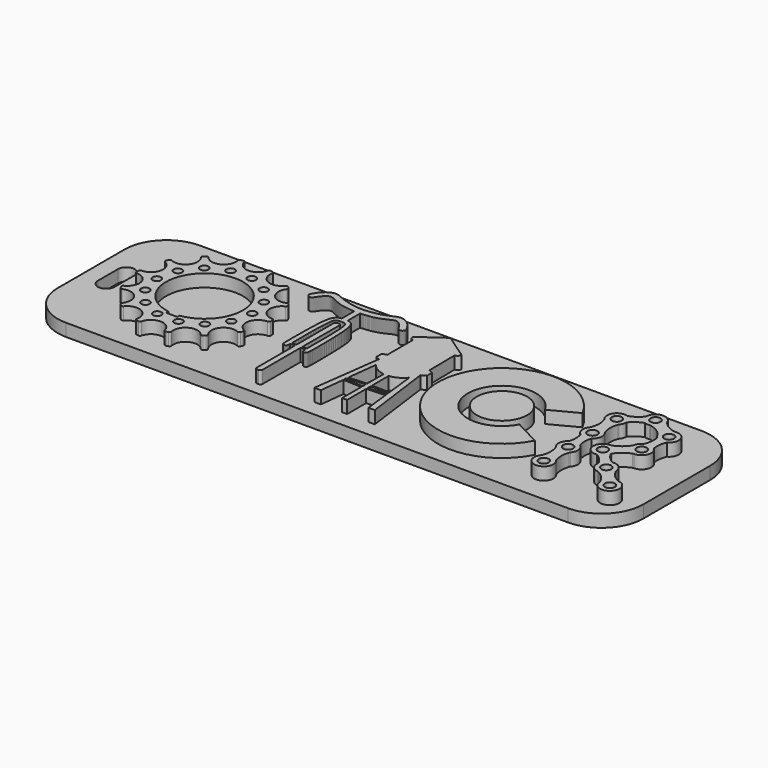
from build123d import *

# Parameters (mm, degrees)
F0_R     = 0.7946644
F1_DEPTH = 2.38125
F0_R_2   = 4.775327
F0_R_3   = 0.9406128
F2_W     = 111.125
F2_H     = 31.75
F3_DEPTH = 2.38125
F4_R     = 7.9375


# Not quite as in the source:
# - ends of sketch curves that miss each other by under 0.0002 mm in the source are joined


with BuildPart() as f1:
    # F0 (on Top) → F1 (new body)
    with BuildSketch(Plane.XY):
        with BuildLine():
            ThreePointArc((-33.590121634, 12.3507484588), (-33.6294176049, 12.5881754555), (-33.8237599562, 12.7301148883))
            ThreePointArc((-33.8237599562, 12.7301148883), (-34.0524121873, 12.7845207856), (-34.2820284084, 12.8347024108))
            ThreePointArc((-34.2820284084, 12.8347024108), (-34.5186909947, 12.7911373675), (-34.6571006347, 12.5942839271))
            ThreePointArc((-34.6571006347, 12.5942839271), (-36.8834641683, 10.8196634), (-39.1098143955, 12.5942824563))
            ThreePointArc((-39.1098143955, 12.5942824563), (-39.2482176053, 12.7911373675), (-39.4848817783, 12.8347100044))
            ThreePointArc((-39.4848817783, 12.8347100044), (-39.7145096927, 12.7845235519), (-39.9431718443, 12.7301060129))
            ThreePointArc((-39.9431718443, 12.7301060129), (-40.1374959801, 12.588167361), (-40.1767882188, 12.3507539588))
            ThreePointArc((-40.1767882188, 12.3507539588), (-41.4126795487, 9.7859172011), (-44.1885186964, 10.4188115386))
            ThreePointArc((-44.1885186964, 10.4188115386), (-44.3986514992, 10.5361025158), (-44.6307849214, 10.4726580069))
            ThreePointArc((-44.6307849214, 10.4726580069), (-44.8158899503, 10.3278331325), (-44.9982810167, 10.1796047146))
            ThreePointArc((-44.9982810167, 10.1796047146), (-45.1117808241, 9.9673948786), (-45.0441752505, 9.7364351367))
            ThreePointArc((-45.0441752505, 9.7364351367), (-45.0448396583, 6.8893584849), (-47.8203948412, 6.2551970986))
            ThreePointArc((-47.8203948412, 6.2551970986), (-48.0606127411, 6.2697127824), (-48.242238874, 6.1118337222))
            ThreePointArc((-48.242238874, 6.1118337222), (-48.3461595976, 5.9010204757), (-48.4461774197, 5.6883278976))
            ThreePointArc((-48.4461774197, 5.6883278976), (-48.4563582226, 5.4478968636), (-48.2952461097, 5.2691472525))
            ThreePointArc((-48.2952461097, 5.2691472525), (-47.0605440786, 2.7037326004), (-49.2860584001, 0.9280908492))
            ThreePointArc((-49.2860584001, 0.9280908492), (-49.5087779976, 0.8369447193), (-49.6039106856, 0.6158986702))
            ThreePointArc((-49.6039106856, 0.6158986702), (-49.6060984, 0.380873), (-49.6039273899, 0.1458470219))
            ThreePointArc((-49.6039273899, 0.1458470219), (-49.5087779976, -0.0751987193), (-49.2860584, -0.1663445635))
            ThreePointArc((-49.2860584, -0.1663445635), (-47.0605440786, -1.9419866004), (-48.2952490252, -4.507395207))
            ThreePointArc((-48.2952490252, -4.507395207), (-48.4563582226, -4.6861508636), (-48.4461664662, -4.9265768698))
            ThreePointArc((-48.4461664662, -4.9265768698), (-48.3461595976, -5.1392744757), (-48.2422297671, -5.3500831279))
            ThreePointArc((-48.2422297671, -5.3500831279), (-48.0606127411, -5.5079667824), (-47.8203983996, -5.4934437005))
            ThreePointArc((-47.8203983996, -5.4934437005), (-45.0448396583, -6.1276124849), (-45.0441705492, -8.9746928823))
            ThreePointArc((-45.0441705492, -8.9746928823), (-45.1117808241, -9.2056488786), (-44.9982729443, -9.4178489662))
            ThreePointArc((-44.9982729443, -9.4178489662), (-44.8158899503, -9.5660871325), (-44.6307918654, -9.7109210511))
            ThreePointArc((-44.6307918654, -9.7109210511), (-44.3986514992, -9.7743565158), (-44.1885265788, -9.6570592469))
            ThreePointArc((-44.1885265788, -9.6570592469), (-41.4126773347, -9.0241468673), (-40.1767873331, -11.5890081606))
            ThreePointArc((-40.1767873331, -11.5890081606), (-40.1374959801, -11.826421361), (-39.9431725738, -11.9683629594))
            ThreePointArc((-39.9431725738, -11.9683629594), (-39.7145096927, -12.0227775519), (-39.4848812536, -12.0729614947))
            ThreePointArc((-39.4848812536, -12.0729614947), (-39.2482176053, -12.0293913675), (-39.1098079653, -11.8325379271))
            ThreePointArc((-39.1098079653, -11.8325379271), (-36.8834641683, -10.0579174), (-34.6571183418, -11.8325419771))
            ThreePointArc((-34.6571183418, -11.8325419771), (-34.5186909947, -12.0293913675), (-34.2820268217, -12.0729640044))
            ThreePointArc((-34.2820268217, -12.0729640044), (-34.0524121873, -12.0227747856), (-33.8237621557, -11.9683600129))
            ThreePointArc((-33.8237621557, -11.9683600129), (-33.6294176049, -11.8264294555), (-33.590121634, -11.5890024588))
            ThreePointArc((-33.590121634, -11.5890024588), (-32.3542358625, -9.0241490812), (-29.5783874048, -9.657043269))
            ThreePointArc((-29.5783874048, -9.657043269), (-29.3682749652, -9.77435434), (-29.1361396594, -9.7109242752))
            ThreePointArc((-29.1361396594, -9.7109242752), (-28.9510364024, -9.566081034), (-28.7686379166, -9.4178462371))
            ThreePointArc((-28.7686379166, -9.4178462371), (-28.6551277759, -9.2056488786), (-28.7227333495, -8.9746891367))
            ThreePointArc((-28.7227333495, -8.9746891367), (-28.7220760775, -6.1276214327), (-25.9465343862, -5.4934411767))
            ThreePointArc((-25.9465343862, -5.4934411767), (-25.7063158426, -5.5079649417), (-25.5246899728, -5.3500775075))
            ThreePointArc((-25.5246899728, -5.3500775075), (-25.4207696215, -5.1392645481), (-25.32075216, -4.9265722676))
            ThreePointArc((-25.32075216, -4.9265722676), (-25.3105542527, -4.6861401007), (-25.4716830986, -4.5073913165))
            ThreePointArc((-25.4716830986, -4.5073913165), (-26.7063870953, -1.9419742188), (-24.4808501999, -0.1663448374))
            ThreePointArc((-24.4808501999, -0.1663448374), (-24.2581307695, -0.0751988834), (-24.162997923, 0.1458468613))
            ThreePointArc((-24.162997923, 0.1458468613), (-24.1608356, 0.380873), (-24.1630066101, 0.6158989781))
            ThreePointArc((-24.1630066101, 0.6158989781), (-24.2581307695, 0.8369448834), (-24.4808502, 0.9280905635))
            ThreePointArc((-24.4808502, 0.9280905635), (-26.7063870953, 2.7037202188), (-25.4716849748, 5.269141207))
            ThreePointArc((-25.4716849748, 5.269141207), (-25.3105542527, 5.4478861007), (-25.3207421338, 5.6883228698))
            ThreePointArc((-25.3207421338, 5.6883228698), (-25.4207696215, 5.9010105481), (-25.524699079, 6.1118189129))
            ThreePointArc((-25.524699079, 6.1118189129), (-25.7063158426, 6.2697109417), (-25.9465356004, 6.2551897005))
            ThreePointArc((-25.9465356004, 6.2551897005), (-28.7220760775, 6.8893674327), (-28.7227380508, 9.7364388823))
            ThreePointArc((-28.7227380508, 9.7364388823), (-28.6551277759, 9.9673948786), (-28.7686356557, 10.1795949662))
            ThreePointArc((-28.7686356557, 10.1795949662), (-28.9510364024, 10.327827034), (-29.1361421346, 10.4726670511))
            ThreePointArc((-29.1361421346, 10.4726670511), (-29.3682749652, 10.53610034), (-29.5783919067, 10.4187928628))
            ThreePointArc((-29.5783919067, 10.4187928628), (-32.3542336486, 9.785919415), (-33.590121634, 12.3507484588))
        make_face()
        with Locations((-38.8217918, -8.4056474)):
            Circle(F0_R, mode=Mode.SUBTRACT)
        with Locations((-42.4421554, -6.6945002)):
            Circle(F0_R, mode=Mode.SUBTRACT)
        with Locations((-34.8175072, -8.3765136)):
            Circle(F0_R, mode=Mode.SUBTRACT)
        with Locations((-31.2224166, -6.61289)):
            Circle(F0_R, mode=Mode.SUBTRACT)
        with Locations((-44.961556, -3.5819842)):
            Circle(F0_R, mode=Mode.SUBTRACT)
        with Locations((-28.7485582, -3.464052)):
            Circle(F0_R, mode=Mode.SUBTRACT)
        with Locations((-45.8809852, 0.3154172)):
            Circle(F0_R, mode=Mode.SUBTRACT)
        with BuildLine():
            ThreePointArc((-37.9286029944, -6.8447817713), (-36.883467, 7.681722), (-35.8383310056, -6.8447817713))
            Line((-35.8383310056, -6.8447817713), (-35.8383332, -7.3637648))
            Line((-35.8383332, -7.3637648), (-37.9286008, -7.3637648))
            Line((-37.9286008, -7.3637648), (-37.9286029944, -6.8447817713))
        make_face(mode=Mode.SUBTRACT)
        with Locations((-27.8859234, 0.4463288)):
            Circle(F0_R, mode=Mode.SUBTRACT)
        with Locations((-45.0183504, 4.225798)):
            Circle(F0_R, mode=Mode.SUBTRACT)
        with Locations((-28.8053526, 4.3437302)):
            Circle(F0_R, mode=Mode.SUBTRACT)
        with Locations((-42.544492, 7.374636)):
            Circle(F0_R, mode=Mode.SUBTRACT)
        with Locations((-38.9494014, 9.1382596)):
            Circle(F0_R, mode=Mode.SUBTRACT)
        with Locations((-31.3247532, 7.4562462)):
            Circle(F0_R, mode=Mode.SUBTRACT)
        with Locations((-34.9451168, 9.1673934)):
            Circle(F0_R, mode=Mode.SUBTRACT)
    extrude(amount=F1_DEPTH)



with BuildPart() as f1b:
    # F0 (on Top) → F1, piece 2 (new body)
    with BuildSketch(Plane.XY):
        with Locations((19.5524374, 0.380873)):
            Circle(F0_R_2)
    extrude(amount=F1_DEPTH)


with BuildPart() as f1c:
    # F0 (on Top) → F1, piece 3 (new body)
    with BuildSketch(Plane.XY):
        with BuildLine():
            ThreePointArc((25.2826844358, -2.633348701), (13.0777742, 0.380873), (25.2826844358, 3.395094701))
            Line((25.2826844358, 3.395094701), (30.3119282, 6.0406026))
            ThreePointArc((30.3119282, 6.0406026), (7.3951592, 0.380873), (30.3119366377, -5.2788610384))
            Line((30.3119366377, -5.2788610384), (25.2826844358, -2.633348701))
        make_face()
    extrude(amount=F1_DEPTH)


with BuildPart() as f1d:
    # F0 (on Top) → F1, piece 4 (new body)
    with BuildSketch(Plane.XY):
        with BuildLine():
            Line((4.4645834, -12.4356114), (5.679186, -12.4356114))
            Line((5.679186, -12.4356114), (3.958463, 0.54991))
            ThreePointArc((3.958463, 0.54991), (4.4173192561, 0.7397615753), (4.8236809314, 1.0251781026))
            Line((4.8236809314, 1.0251781026), (4.8493426, 2.198497))
            ThreePointArc((4.8493426, 2.198497), (4.4533409594, 2.4265248649), (4.0170864794, 2.5625312363))
            Line((4.0170864794, 2.5625312363), (3.941191, 8.6607142))
            ThreePointArc((3.941191, 8.6607142), (4.4449083132, 8.8954168394), (4.7161825983, 9.380420758))
            Line((4.7161825983, 9.380420758), (-0.0563372, 12.6585726))
            Line((-0.0563372, 12.6585726), (-4.574159, 9.4512384))
            ThreePointArc((-4.574159, 9.4512384), (-4.4374640474, 8.9238193385), (-3.9651421172, 8.6522138729))
            Line((-3.9651421172, 8.6522138729), (-3.959479, 2.5776174))
            ThreePointArc((-3.959479, 2.5776174), (-4.4068158157, 2.4445470258), (-4.8173908735, 2.2226291598))
            Line((-4.8173908735, 2.2226291598), (-4.7921164, 1.0034524))
            ThreePointArc((-4.7921164, 1.0034524), (-4.4323052844, 0.8270572106), (-4.0505879444, 0.7051075587))
            Line((-4.0505879444, 0.7051075587), (-5.7918858, -12.4356114))
            Line((-5.7918858, -12.4356114), (-4.5598334, -12.4356114))
            Line((-4.5598334, -12.4356114), (-4.0266874, -7.7761592))
            Line((-4.0266874, -7.7761592), (-0.5179314, -7.8915768))
            Line((-0.5179314, -7.8915768), (-0.5179314, -12.4356114))
            Line((-0.5179314, -12.4356114), (0.4226814, -12.4356114))
            Line((0.4226814, -12.4356114), (0.4226814, -7.9140812))
            Line((0.4226814, -7.9140812), (3.9224204, -7.6973938))
            Line((3.9224204, -7.6973938), (4.4645834, -12.4356114))
        make_face()
        Polygon((-0.5179314, -6.8287392), (-0.5179314, -7.5406758), (-4.0517318, -7.4238612), (-3.9769542, -7.088886), align=None, mode=Mode.SUBTRACT)
        with BuildLine():
            Line((-0.5179314, -6.4943736), (-3.9253668, -6.7382136))
            Line((-3.9253668, -6.7382136), (-3.2671258, -0.985393))
            ThreePointArc((-3.2671258, -0.985393), (-2.0560803671, -2.0688932492), (-0.5179318251, -2.5930131115))
            Line((-0.5179318251, -2.5930131115), (-0.5179314, -6.4943736))
        make_face(mode=Mode.SUBTRACT)
        Polygon((3.7990018, -7.0056756), (3.8354254, -7.323963), (0.4226814, -7.5932538), (0.4226814, -6.895592), align=None, mode=Mode.SUBTRACT)
        with BuildLine():
            Line((3.1691326, -1.1139932), (3.8027356, -6.6512186))
            Line((3.8027356, -6.6512186), (0.4226814, -6.5249552))
            Line((0.4226814, -6.5249552), (0.4226814, -2.6042874))
            ThreePointArc((0.4226814, -2.6042874), (1.9444372298, -2.1328635042), (3.1691326, -1.1139932))
        make_face(mode=Mode.SUBTRACT)
    extrude(amount=F1_DEPTH)


with BuildPart() as f1e:
    # F0 (on Top) → F1, piece 5 (new body)
    with BuildSketch(Plane.XY):
        with BuildLine():
            Line((-15.9458914, 11.6212112), (-15.9545528, 11.6212112))
            Line((-15.9545528, 11.6212112), (-16.547592, 11.655298))
            Line((-16.547592, 11.655298), (-17.088739, 11.705336))
            Line((-17.088739, 11.705336), (-17.581626, 11.768836))
            Line((-17.581626, 11.768836), (-18.0299106, 11.8433596))
            Line((-18.0299106, 11.8433596), (-18.437225, 11.9264938))
            Line((-18.437225, 11.9264938), (-18.8072268, 12.0157748))
            Line((-18.8072268, 12.0157748), (-19.1435482, 12.1087896))
            Line((-19.1435482, 12.1087896), (-19.4498214, 12.203049))
            Line((-19.4498214, 12.203049), (-19.7293738, 12.2964194))
            Line((-19.7293738, 12.2964194), (-19.9841612, 12.3877832))
            Line((-19.9841612, 12.3877832), (-20.215733, 12.4762514))
            Line((-20.215733, 12.4762514), (-20.4257656, 12.5610112))
            Line((-20.4257656, 12.5610112), (-20.6158338, 12.641199))
            Line((-20.6158338, 12.641199), (-20.7875378, 12.7159258))
            Line((-20.7875378, 12.7159258), (-20.9425286, 12.7843788))
            Line((-20.9425286, 12.7843788), (-21.082381, 12.8456944))
            Line((-21.082381, 12.8456944), (-21.2086952, 12.8992376))
            Line((-21.2086952, 12.8992376), (-21.3230968, 12.9454148))
            Line((-21.3230968, 12.9454148), (-21.4272114, 12.9848102))
            Line((-21.4272114, 12.9848102), (-21.5226392, 13.0180334))
            Line((-21.5226392, 13.0180334), (-21.6109804, 13.0457194))
            Line((-21.6109804, 13.0457194), (-21.6938606, 13.0684524))
            Line((-21.6938606, 13.0684524), (-21.77288, 13.0868674))
            Line((-21.77288, 13.0868674), (-21.8496388, 13.1015232))
            Line((-21.8496388, 13.1015232), (-21.925534, 13.1129786))
            Line((-21.925534, 13.1129786), (-22.001099, 13.1212844))
            Line((-22.001099, 13.1212844), (-22.0765878, 13.126339))
            Line((-22.0765878, 13.126339), (-22.1522798, 13.1281424))
            Line((-22.1522798, 13.1281424), (-22.2284544, 13.1266184))
            Line((-22.2284544, 13.1266184), (-22.3054418, 13.1216908))
            Line((-22.3054418, 13.1216908), (-22.3834706, 13.1133596))
            Line((-22.3834706, 13.1133596), (-22.4628456, 13.1015232))
            Line((-22.4628456, 13.1015232), (-22.54377, 13.0861562))
            Line((-22.54377, 13.0861562), (-22.6261168, 13.067157))
            Line((-22.6261168, 13.067157), (-22.7096828, 13.044424))
            Line((-22.7096828, 13.044424), (-22.7942648, 13.0178556))
            Line((-22.7942648, 13.0178556), (-22.8796596, 12.9873502))
            Line((-22.8796596, 12.9873502), (-22.9656894, 12.9528316))
            Line((-22.9656894, 12.9528316), (-23.0521002, 12.9141982))
            Line((-23.0521002, 12.9141982), (-23.1387142, 12.8713484))
            Line((-23.1387142, 12.8713484), (-23.2253536, 12.8242314))
            Line((-23.2253536, 12.8242314), (-23.3117898, 12.7730504))
            Line((-23.3117898, 12.7730504), (-23.3978196, 12.7180594))
            Line((-23.3978196, 12.7180594), (-23.4832906, 12.6595124))
            Line((-23.4832906, 12.6595124), (-23.5679996, 12.5976634))
            Line((-23.5679996, 12.5976634), (-23.6517688, 12.5327664))
            Line((-23.6517688, 12.5327664), (-23.7343696, 12.4650754))
            Line((-23.7343696, 12.4650754), (-23.8156242, 12.3948444))
            Line((-23.8156242, 12.3948444), (-23.895431, 12.322175))
            Line((-23.895431, 12.322175), (-23.9741456, 12.246483))
            Line((-23.9741456, 12.246483), (-24.0521744, 12.1670572))
            Line((-24.0521744, 12.1670572), (-24.1298984, 12.0832372))
            Line((-24.1298984, 12.0832372), (-24.2077494, 11.994261))
            Line((-24.2077494, 11.994261), (-24.2861846, 11.8994174))
            Line((-24.2861846, 11.8994174), (-24.3655596, 11.7980206))
            Line((-24.3655596, 11.7980206), (-24.446357, 11.689334))
            Line((-24.446357, 11.689334), (-24.5286022, 11.5731798))
            Line((-24.5286022, 11.5731798), (-24.610949, 11.4514884))
            Line((-24.610949, 11.4514884), (-24.6917718, 11.3267236))
            Line((-24.6917718, 11.3267236), (-24.7693688, 11.2014))
            Line((-24.7693688, 11.2014), (-24.842089, 11.0779052))
            Line((-24.842089, 11.0779052), (-24.9082052, 10.9587792))
            Line((-24.9082052, 10.9587792), (-24.9660664, 10.846435))
            Line((-24.9660664, 10.846435), (-25.0140216, 10.7433872))
            Line((-25.0140216, 10.7433872), (-25.0508008, 10.6514138))
            Line((-25.0508008, 10.6514138), (-25.0768866, 10.5699052))
            Line((-25.0768866, 10.5699052), (-25.093168, 10.4975406))
            Line((-25.093168, 10.4975406), (-25.1005848, 10.4329992))
            Line((-25.1005848, 10.4329992), (-25.100026, 10.3750364))
            Line((-25.100026, 10.3750364), (-25.092406, 10.3222806))
            Line((-25.092406, 10.3222806), (-25.0786138, 10.2735126))
            Line((-25.0786138, 10.2735126), (-25.0595892, 10.2273608))
            Line((-25.0595892, 10.2273608), (-25.0361196, 10.18286))
            Line((-25.0361196, 10.18286), (-25.0086368, 10.1401118))
            Line((-25.0086368, 10.1401118), (-24.977471, 10.0994718))
            Line((-24.977471, 10.0994718), (-24.942927, 10.0613718))
            Line((-24.942927, 10.0613718), (-24.9053858, 10.0261928))
            Line((-24.9053858, 10.0261928), (-24.8651522, 9.9943158))
            Line((-24.8651522, 9.9943158), (-24.822531, 9.9661218))
            Line((-24.822531, 9.9661218), (-24.7778778, 9.9420426))
            Line((-24.7778778, 9.9420426), (-24.7315482, 9.9223576))
            Line((-24.7315482, 9.9223576), (-24.6839232, 9.9069652))
            Line((-24.6839232, 9.9069652), (-24.6354346, 9.8957638))
            Line((-24.6354346, 9.8957638), (-24.5865396, 9.8885502))
            Line((-24.5865396, 9.8885502), (-24.5376446, 9.885172))
            Line((-24.5376446, 9.885172), (-24.489156, 9.8854768))
            Line((-24.489156, 9.8854768), (-24.441531, 9.8893122))
            Line((-24.441531, 9.8893122), (-24.3952014, 9.8965258))
            Line((-24.3952014, 9.8965258), (-24.3504466, 9.907016))
            Line((-24.3504466, 9.907016), (-24.3070888, 9.9211638))
            Line((-24.3070888, 9.9211638), (-24.2647978, 9.9393756))
            Line((-24.2647978, 9.9393756), (-24.2233196, 9.9621594))
            Line((-24.2233196, 9.9621594), (-24.1822732, 9.9898962))
            Line((-24.1822732, 9.9898962), (-24.1413792, 10.0230686))
            Line((-24.1413792, 10.0230686), (-24.1003328, 10.0621084))
            Line((-24.1003328, 10.0621084), (-24.0588292, 10.1074728))
            Line((-24.0588292, 10.1074728), (-24.0165128, 10.1594412))
            Line((-24.0165128, 10.1594412), (-23.9730026, 10.2177088))
            Line((-23.9730026, 10.2177088), (-23.927943, 10.2818184))
            Line((-23.927943, 10.2818184), (-23.8808768, 10.3513382))
            Line((-23.8808768, 10.3513382), (-23.831423, 10.425811))
            Line((-23.831423, 10.425811), (-23.7791752, 10.5047542))
            Line((-23.7791752, 10.5047542), (-23.7237524, 10.587736))
            Line((-23.7237524, 10.587736), (-23.6647482, 10.6743246))
            Line((-23.6647482, 10.6743246), (-23.6019086, 10.7639104))
            Line((-23.6019086, 10.7639104), (-23.5355638, 10.8555536))
            Line((-23.5355638, 10.8555536), (-23.466171, 10.9481366))
            Line((-23.466171, 10.9481366), (-23.3942382, 11.0405418))
            Line((-23.3942382, 11.0405418), (-23.3202734, 11.1317278))
            Line((-23.3202734, 11.1317278), (-23.244683, 11.220577))
            Line((-23.244683, 11.220577), (-23.1680258, 11.3059718))
            Line((-23.1680258, 11.3059718), (-23.0907082, 11.3868708))
            Line((-23.0907082, 11.3868708), (-23.0132636, 11.4622834))
            Line((-23.0132636, 11.4622834), (-22.936073, 11.531981))
            Line((-22.936073, 11.531981), (-22.859492, 11.5957858))
            Line((-22.859492, 11.5957858), (-22.7839524, 11.6535962))
            Line((-22.7839524, 11.6535962), (-22.7098606, 11.7052852))
            Line((-22.7098606, 11.7052852), (-22.6375722, 11.7507512))
            Line((-22.6375722, 11.7507512), (-22.5674682, 11.7898418))
            Line((-22.5674682, 11.7898418), (-22.4999804, 11.82243))
            Line((-22.4999804, 11.82243), (-22.4353374, 11.8485158))
            Line((-22.4353374, 11.8485158), (-22.3732598, 11.8685056))
            Line((-22.3732598, 11.8685056), (-22.3132904, 11.882882))
            Line((-22.3132904, 11.882882), (-22.2550228, 11.892153))
            Line((-22.2550228, 11.892153), (-22.1979744, 11.896852))
            Line((-22.1979744, 11.896852), (-22.1417388, 11.8974616))
            Line((-22.1417388, 11.8974616), (-22.0858842, 11.8944898))
            Line((-22.0858842, 11.8944898), (-22.0299788, 11.8884446))
            Line((-22.0299788, 11.8884446), (-21.9734384, 11.879707))
            Line((-21.9734384, 11.879707), (-21.915247, 11.8679214))
            Line((-21.915247, 11.8679214), (-21.8542616, 11.8527068))
            Line((-21.8542616, 11.8527068), (-21.7892884, 11.8335298))
            Line((-21.7892884, 11.8335298), (-21.7191844, 11.8100094))
            Line((-21.7191844, 11.8100094), (-21.6428066, 11.7816376))
            Line((-21.6428066, 11.7816376), (-21.5589866, 11.7479826))
            Line((-21.5589866, 11.7479826), (-21.4665814, 11.7086126))
            Line((-21.4665814, 11.7086126), (-21.3648036, 11.6632736))
            Line((-21.3648036, 11.6632736), (-21.2544152, 11.6127022))
            Line((-21.2544152, 11.6127022), (-21.13661, 11.5578382))
            Line((-21.13661, 11.5578382), (-21.012531, 11.4996468))
            Line((-21.012531, 11.4996468), (-20.8832958, 11.4390678))
            Line((-20.8832958, 11.4390678), (-20.7500982, 11.3770664))
            Line((-20.7500982, 11.3770664), (-20.6141066, 11.3145824))
            Line((-20.6141066, 11.3145824), (-20.476464, 11.2525556))
            Line((-20.476464, 11.2525556), (-20.3380848, 11.1918242))
            Line((-20.3380848, 11.1918242), (-20.1990706, 11.1327184))
            Line((-20.1990706, 11.1327184), (-20.059269, 11.0754414))
            Line((-20.059269, 11.0754414), (-19.9185022, 11.020171))
            Line((-19.9185022, 11.020171), (-19.7766686, 10.9671358))
            Line((-19.7766686, 10.9671358), (-19.6336158, 10.9164882))
            Line((-19.6336158, 10.9164882), (-19.489166, 10.8684568))
            Line((-19.489166, 10.8684568), (-19.3431922, 10.8232194))
            Line((-19.3431922, 10.8232194), (-19.1953388, 10.7809284))
            Line((-19.1953388, 10.7809284), (-19.0444628, 10.741406))
            Line((-19.0444628, 10.741406), (-18.8891926, 10.7044236))
            Line((-18.8891926, 10.7044236), (-18.7282328, 10.669778))
            Line((-18.7282328, 10.669778), (-18.560161, 10.6372152))
            Line((-18.560161, 10.6372152), (-18.3836564, 10.606532))
            Line((-18.3836564, 10.606532), (-18.1973982, 10.577449))
            Line((-18.1973982, 10.577449), (-17.9999894, 10.5497884))
            Line((-17.9999894, 10.5497884), (-17.7913538, 10.5234486))
            Line((-17.7913538, 10.5234486), (-17.5765206, 10.4987852))
            Line((-17.5765206, 10.4987852), (-17.3617382, 10.4763316))
            Line((-17.3617382, 10.4763316), (-17.1533058, 10.4565958))
            Line((-17.1533058, 10.4565958), (-16.9574464, 10.4400858))
            Line((-16.9574464, 10.4400858), (-16.7804846, 10.4273096))
            Line((-16.7804846, 10.4273096), (-16.6286688, 10.418826))
            Line((-16.6286688, 10.418826), (-16.5082728, 10.4150922))
            Line((-16.5082728, 10.4150922), (-16.5082728, 7.4820272))
            Line((-16.5082728, 7.4820272), (-16.7950134, 7.4200004))
            Line((-16.7950134, 7.4200004), (-16.8914318, 7.39267))
            Line((-16.8914318, 7.39267), (-16.9828464, 7.3597262))
            Line((-16.9828464, 7.3597262), (-17.0701462, 7.3207118))
            Line((-17.0701462, 7.3207118), (-17.1541948, 7.2752458))
            Line((-17.1541948, 7.2752458), (-17.235805, 7.2228456))
            Line((-17.235805, 7.2228456), (-17.315688, 7.1629778))
            Line((-17.315688, 7.1629778), (-17.3937168, 7.0945248))
            Line((-17.3937168, 7.0945248), (-17.4696374, 7.0162166))
            Line((-17.4696374, 7.0162166), (-17.5430942, 6.9267578))
            Line((-17.5430942, 6.9267578), (-17.6138586, 6.8249292))
            Line((-17.6138586, 6.8249292), (-17.6816258, 6.7094354))
            Line((-17.6816258, 6.7094354), (-17.746091, 6.5790318))
            Line((-17.746091, 6.5790318), (-17.8069494, 6.4324484))
            Line((-17.8069494, 6.4324484), (-17.8639978, 6.2680596))
            Line((-17.8639978, 6.2680596), (-17.9172108, 6.0828428))
            Line((-17.9172108, 6.0828428), (-17.9666392, 5.8734452))
            Line((-17.9666392, 5.8734452), (-18.0123592, 5.636514))
            Line((-18.0123592, 5.636514), (-18.0544216, 5.368671))
            Line((-18.0544216, 5.368671), (-18.0928518, 5.066538))
            Line((-18.0928518, 5.066538), (-18.1277006, 4.7267622))
            Line((-18.1277006, 4.7267622), (-18.1590696, 4.3459908))
            Line((-18.1590696, 4.3459908), (-18.1869842, 3.922395))
            Line((-18.1869842, 3.922395), (-18.2116476, 3.4605722))
            Line((-18.2116476, 3.4605722), (-18.2332884, 2.9666692))
            Line((-18.2332884, 2.9666692), (-18.2521098, 2.446782))
            Line((-18.2521098, 2.446782), (-18.2683404, 1.9070574))
            Line((-18.2683404, 1.9070574), (-18.2822088, 1.3536676))
            Line((-18.2822088, 1.3536676), (-18.2938928, 0.792734))
            Line((-18.2938928, 0.792734), (-18.3036464, 0.230378))
            Line((-18.3036464, 0.230378), (-18.3115966, -0.3270504))
            Line((-18.3115966, -0.3270504), (-18.3177434, -0.8723884))
            Line((-18.3177434, -0.8723884), (-18.3219598, -1.3982954))
            Line((-18.3219598, -1.3982954), (-18.3241188, -1.8974308))
            Line((-18.3241188, -1.8974308), (-18.3241696, -2.3624286))
            Line((-18.3241696, -2.3624286), (-18.3219852, -2.7859482))
            Line((-18.3219852, -2.7859482), (-18.317464, -3.1605982))
            Line((-18.317464, -3.1605982), (-18.3105044, -3.4790888))
            Line((-18.3105044, -3.4790888), (-18.3010302, -3.7365178))
            Line((-18.3010302, -3.7365178), (-18.2889398, -3.938016))
            Line((-18.2889398, -3.938016), (-18.274157, -4.0912542))
            Line((-18.274157, -4.0912542), (-18.2566056, -4.2038016))
            Line((-18.2566056, -4.2038016), (-18.2362348, -4.283329))
            Line((-18.2362348, -4.283329), (-18.2129684, -4.3374564))
            Line((-18.2129684, -4.3374564), (-18.1866794, -4.3737784))
            Line((-18.1866794, -4.3737784), (-18.1573678, -4.3999404))
            Line((-18.1573678, -4.3999404), (-18.1249828, -4.4222924))
            Line((-18.1249828, -4.4222924), (-18.08988, -4.4420536))
            Line((-18.08988, -4.4420536), (-18.0524912, -4.4591224))
            Line((-18.0524912, -4.4591224), (-18.0132228, -4.4734226))
            Line((-18.0132228, -4.4734226), (-17.9725066, -4.484878))
            Line((-17.9725066, -4.484878), (-17.9307744, -4.4934632))
            Line((-17.9307744, -4.4934632), (-17.888458, -4.4990258))
            Line((-17.888458, -4.4990258), (-17.8459384, -4.5015404))
            Line((-17.8459384, -4.5015404), (-17.803622, -4.5009562))
            Line((-17.803622, -4.5009562), (-17.7618136, -4.4972732))
            Line((-17.7618136, -4.4972732), (-17.7207672, -4.4905422))
            Line((-17.7207672, -4.4905422), (-17.6807114, -4.480814))
            Line((-17.6807114, -4.480814), (-17.641951, -4.4681394))
            Line((-17.641951, -4.4681394), (-17.6046892, -4.4525438))
            Line((-17.6046892, -4.4525438), (-17.5692308, -4.434078))
            Line((-17.5692308, -4.434078), (-17.535779, -4.4128182))
            Line((-17.535779, -4.4128182), (-17.5046386, -4.3870118))
            Line((-17.5046386, -4.3870118), (-17.4760382, -4.3478958))
            Line((-17.4760382, -4.3478958), (-17.4502572, -4.2850054))
            Line((-17.4502572, -4.2850054), (-17.427575, -4.1877742))
            Line((-17.427575, -4.1877742), (-17.4081948, -4.0456866))
            Line((-17.4081948, -4.0456866), (-17.3924214, -3.8482524))
            Line((-17.3924214, -3.8482524), (-17.385538, -3.6964874))
            Line((-17.385538, -3.6964874), (-16.5025578, -3.6964874))
            Line((-16.5025578, -3.6964874), (-16.5025578, -12.681331))
            ThreePointArc((-16.5025578, -12.681331), (-16.3716718103, -12.9972564103), (-16.0557464, -13.128117))
            Line((-16.0557464, -13.128117), (-15.9502094, -13.128117))
            Line((-15.9502094, -13.128117), (-15.8446724, -13.128117))
            ThreePointArc((-15.8446724, -13.128117), (-15.5287469897, -12.9972564103), (-15.3978864, -12.681331))
            Line((-15.3978864, -12.681331), (-15.3978864, -3.6964874))
            Line((-15.3978864, -3.6964874), (-14.5149062, -3.6964874))
            Line((-14.5149062, -3.6964874), (-14.5080228, -3.8482524))
            Line((-14.5080228, -3.8482524), (-14.4922494, -4.0456866))
            Line((-14.4922494, -4.0456866), (-14.4728692, -4.1877742))
            Line((-14.4728692, -4.1877742), (-14.4501616, -4.2850054))
            Line((-14.4501616, -4.2850054), (-14.4243806, -4.3478958))
            Line((-14.4243806, -4.3478958), (-14.3958056, -4.3870118))
            Line((-14.3958056, -4.3870118), (-14.3646398, -4.4128182))
            Line((-14.3646398, -4.4128182), (-14.3312134, -4.434078))
            Line((-14.3312134, -4.434078), (-14.2957296, -4.4525438))
            Line((-14.2957296, -4.4525438), (-14.2584932, -4.4681394))
            Line((-14.2584932, -4.4681394), (-14.2197074, -4.480814))
            Line((-14.2197074, -4.480814), (-14.179677, -4.4905422))
            Line((-14.179677, -4.4905422), (-14.1386052, -4.4972732))
            Line((-14.1386052, -4.4972732), (-14.0968222, -4.5009562))
            Line((-14.0968222, -4.5009562), (-14.0545058, -4.5015404))
            Line((-14.0545058, -4.5015404), (-14.0119862, -4.4990258))
            Line((-14.0119862, -4.4990258), (-13.9696444, -4.4934632))
            Line((-13.9696444, -4.4934632), (-13.9279122, -4.484878))
            Line((-13.9279122, -4.484878), (-13.887196, -4.4734226))
            Line((-13.887196, -4.4734226), (-13.847953, -4.4591224))
            Line((-13.847953, -4.4591224), (-13.8105642, -4.4420536))
            Line((-13.8105642, -4.4420536), (-13.7754614, -4.4222924))
            Line((-13.7754614, -4.4222924), (-13.7430764, -4.3999404))
            Line((-13.7430764, -4.3999404), (-13.7137394, -4.3737784))
            Line((-13.7137394, -4.3737784), (-13.6874758, -4.3374564))
            Line((-13.6874758, -4.3374564), (-13.664184, -4.283329))
            Line((-13.664184, -4.283329), (-13.6438132, -4.2038016))
            Line((-13.6438132, -4.2038016), (-13.6262872, -4.0912542))
            Line((-13.6262872, -4.0912542), (-13.6115044, -3.938016))
            Line((-13.6115044, -3.938016), (-13.599414, -3.7365178))
            Line((-13.599414, -3.7365178), (-13.5899398, -3.4790888))
            Line((-13.5899398, -3.4790888), (-13.5829802, -3.1605982))
            Line((-13.5829802, -3.1605982), (-13.578459, -2.7859482))
            Line((-13.578459, -2.7859482), (-13.5762746, -2.3624286))
            Line((-13.5762746, -2.3624286), (-13.5763, -1.8974308))
            Line((-13.5763, -1.8974308), (-13.5784844, -1.3982954))
            Line((-13.5784844, -1.3982954), (-13.5827008, -0.8723884))
            Line((-13.5827008, -0.8723884), (-13.5888222, -0.3270504))
            Line((-13.5888222, -0.3270504), (-13.5967978, 0.230378))
            Line((-13.5967978, 0.230378), (-13.606526, 0.792734))
            Line((-13.606526, 0.792734), (-13.6182354, 1.3536676))
            Line((-13.6182354, 1.3536676), (-13.6320784, 1.9070574))
            Line((-13.6320784, 1.9070574), (-13.648309, 2.446782))
            Line((-13.648309, 2.446782), (-13.6671558, 2.9666692))
            Line((-13.6671558, 2.9666692), (-13.6887966, 3.4605722))
            Line((-13.6887966, 3.4605722), (-13.71346, 3.922395))
            Line((-13.71346, 3.922395), (-13.7413746, 4.3459908))
            Line((-13.7413746, 4.3459908), (-13.7727182, 4.7267622))
            Line((-13.7727182, 4.7267622), (-13.8075924, 5.066538))
            Line((-13.8075924, 5.066538), (-13.8460226, 5.368671))
            Line((-13.8460226, 5.368671), (-13.8880596, 5.636514))
            Line((-13.8880596, 5.636514), (-13.9337796, 5.8734452))
            Line((-13.9337796, 5.8734452), (-13.9832334, 6.0828428))
            Line((-13.9832334, 6.0828428), (-14.0364464, 6.2680596))
            Line((-14.0364464, 6.2680596), (-14.0934948, 6.4324484))
            Line((-14.0934948, 6.4324484), (-14.1543532, 6.5790318))
            Line((-14.1543532, 6.5790318), (-14.2188184, 6.7094354))
            Line((-14.2188184, 6.7094354), (-14.2865602, 6.8249292))
            Line((-14.2865602, 6.8249292), (-14.3573246, 6.9267578))
            Line((-14.3573246, 6.9267578), (-14.4308068, 7.0162166))
            Line((-14.4308068, 7.0162166), (-14.506702, 7.0945248))
            Line((-14.506702, 7.0945248), (-14.5847562, 7.1629778))
            Line((-14.5847562, 7.1629778), (-14.6646138, 7.2228456))
            Line((-14.6646138, 7.2228456), (-14.7462494, 7.2752458))
            Line((-14.7462494, 7.2752458), (-14.8302726, 7.3207118))
            Line((-14.8302726, 7.3207118), (-14.9175724, 7.3597262))
            Line((-14.9175724, 7.3597262), (-15.0090124, 7.39267))
            Line((-15.0090124, 7.39267), (-15.1054308, 7.4200004))
            Line((-15.1054308, 7.4200004), (-15.2076912, 7.4421238))
            Line((-15.2076912, 7.4421238), (-15.3921714, 7.4714862))
            Line((-15.3921714, 7.4714862), (-15.3897076, 10.4151684))
            Line((-15.3897076, 10.4151684), (-15.2701244, 10.4188768))
            Line((-15.2701244, 10.4188768), (-15.1189182, 10.4273604))
            Line((-15.1189182, 10.4273604), (-14.9423882, 10.4400858))
            Line((-14.9423882, 10.4400858), (-14.7468336, 10.4565958))
            Line((-14.7468336, 10.4565958), (-14.5385536, 10.4763316))
            Line((-14.5385536, 10.4763316), (-14.3238728, 10.4987852))
            Line((-14.3238728, 10.4987852), (-14.109065, 10.5234486))
            Line((-14.109065, 10.5234486), (-13.9004548, 10.5497884))
            Line((-13.9004548, 10.5497884), (-13.703046, 10.577449))
            Line((-13.703046, 10.577449), (-13.5167624, 10.606532))
            Line((-13.5167624, 10.606532), (-13.3402832, 10.6372152))
            Line((-13.3402832, 10.6372152), (-13.1722114, 10.669778))
            Line((-13.1722114, 10.669778), (-13.0112262, 10.7044236))
            Line((-13.0112262, 10.7044236), (-12.8559814, 10.741406))
            Line((-12.8559814, 10.741406), (-12.7051054, 10.7809284))
            Line((-12.7051054, 10.7809284), (-12.557252, 10.8232194))
            Line((-12.557252, 10.8232194), (-12.4112782, 10.8684568))
            Line((-12.4112782, 10.8684568), (-12.2668284, 10.9164882))
            Line((-12.2668284, 10.9164882), (-12.1237502, 10.9671358))
            Line((-12.1237502, 10.9671358), (-11.9819166, 11.020171))
            Line((-11.9819166, 11.020171), (-11.8411752, 11.0754414))
            Line((-11.8411752, 11.0754414), (-11.7013736, 11.1327184))
            Line((-11.7013736, 11.1327184), (-11.5623594, 11.1918242))
            Line((-11.5623594, 11.1918242), (-11.4239802, 11.2525556))
            Line((-11.4239802, 11.2525556), (-11.2863376, 11.3145824))
            Line((-11.2863376, 11.3145824), (-11.1503206, 11.3770664))
            Line((-11.1503206, 11.3770664), (-11.0171484, 11.4390678))
            Line((-11.0171484, 11.4390678), (-10.8879132, 11.4996468))
            Line((-10.8879132, 11.4996468), (-10.7638342, 11.5578382))
            Line((-10.7638342, 11.5578382), (-10.6460036, 11.6127022))
            Line((-10.6460036, 11.6127022), (-10.5356406, 11.6632736))
            Line((-10.5356406, 11.6632736), (-10.4338628, 11.7086126))
            Line((-10.4338628, 11.7086126), (-10.3414322, 11.7479826))
            Line((-10.3414322, 11.7479826), (-10.2576376, 11.7816376))
            Line((-10.2576376, 11.7816376), (-10.1812598, 11.8100094))
            Line((-10.1812598, 11.8100094), (-10.1111558, 11.8335298))
            Line((-10.1111558, 11.8335298), (-10.0461826, 11.8527068))
            Line((-10.0461826, 11.8527068), (-9.9851718, 11.8679214))
            Line((-9.9851718, 11.8679214), (-9.9269804, 11.879707))
            Line((-9.9269804, 11.879707), (-9.8704654, 11.8884446))
            Line((-9.8704654, 11.8884446), (-9.8145346, 11.8944898))
            Line((-9.8145346, 11.8944898), (-9.75868, 11.8974616))
            Line((-9.75868, 11.8974616), (-9.7024444, 11.896852))
            Line((-9.7024444, 11.896852), (-9.6454214, 11.892153))
            Line((-9.6454214, 11.892153), (-9.5871284, 11.882882))
            Line((-9.5871284, 11.882882), (-9.527159, 11.8685056))
            Line((-9.527159, 11.8685056), (-9.4650814, 11.8485158))
            Line((-9.4650814, 11.8485158), (-9.4004384, 11.82243))
            Line((-9.4004384, 11.82243), (-9.3329506, 11.7898418))
            Line((-9.3329506, 11.7898418), (-9.262872, 11.7507512))
            Line((-9.262872, 11.7507512), (-9.1905836, 11.7052852))
            Line((-9.1905836, 11.7052852), (-9.1164664, 11.6535962))
            Line((-9.1164664, 11.6535962), (-9.0409268, 11.5957858))
            Line((-9.0409268, 11.5957858), (-8.9643712, 11.531981))
            Line((-8.9643712, 11.531981), (-8.8871806, 11.4622834))
            Line((-8.8871806, 11.4622834), (-8.8097106, 11.3868708))
            Line((-8.8097106, 11.3868708), (-8.7324184, 11.3059718))
            Line((-8.7324184, 11.3059718), (-8.6557358, 11.220577))
            Line((-8.6557358, 11.220577), (-8.5801708, 11.1317278))
            Line((-8.5801708, 11.1317278), (-8.5061806, 11.0405418))
            Line((-8.5061806, 11.0405418), (-8.4342732, 10.9481366))
            Line((-8.4342732, 10.9481366), (-8.3648804, 10.8555536))
            Line((-8.3648804, 10.8555536), (-8.2985356, 10.7639104))
            Line((-8.2985356, 10.7639104), (-8.235696, 10.6743246))
            Line((-8.235696, 10.6743246), (-8.1766664, 10.587736))
            Line((-8.1766664, 10.587736), (-8.1212436, 10.5047542))
            Line((-8.1212436, 10.5047542), (-8.0690212, 10.425811))
            Line((-8.0690212, 10.425811), (-8.0195674, 10.3513382))
            Line((-8.0195674, 10.3513382), (-7.9725012, 10.2818184))
            Line((-7.9725012, 10.2818184), (-7.9274162, 10.2177088))
            Line((-7.9274162, 10.2177088), (-7.8839314, 10.1594412))
            Line((-7.8839314, 10.1594412), (-7.841615, 10.1074728))
            Line((-7.841615, 10.1074728), (-7.800086, 10.0621084))
            Line((-7.800086, 10.0621084), (-7.7590396, 10.0230686))
            Line((-7.7590396, 10.0230686), (-7.718171, 9.9898962))
            Line((-7.718171, 9.9898962), (-7.6771246, 9.9621594))
            Line((-7.6771246, 9.9621594), (-7.635621, 9.9393756))
            Line((-7.635621, 9.9393756), (-7.5933554, 9.9211638))
            Line((-7.5933554, 9.9211638), (-7.5499976, 9.907016))
            Line((-7.5499976, 9.907016), (-7.5052428, 9.8965258))
            Line((-7.5052428, 9.8965258), (-7.4588878, 9.8893122))
            Line((-7.4588878, 9.8893122), (-7.4112882, 9.8854768))
            Line((-7.4112882, 9.8854768), (-7.3627996, 9.885172))
            Line((-7.3627996, 9.885172), (-7.3139046, 9.8885502))
            Line((-7.3139046, 9.8885502), (-7.2649842, 9.8957638))
            Line((-7.2649842, 9.8957638), (-7.216521, 9.9069652))
            Line((-7.216521, 9.9069652), (-7.168896, 9.9223576))
            Line((-7.168896, 9.9223576), (-7.122541, 9.9420426))
            Line((-7.122541, 9.9420426), (-7.0779132, 9.9661218))
            Line((-7.0779132, 9.9661218), (-7.035292, 9.9943158))
            Line((-7.035292, 9.9943158), (-6.9950584, 10.0261928))
            Line((-6.9950584, 10.0261928), (-6.9574918, 10.0613718))
            Line((-6.9574918, 10.0613718), (-6.9229732, 10.0994718))
            Line((-6.9229732, 10.0994718), (-6.8918074, 10.1401118))
            Line((-6.8918074, 10.1401118), (-6.8643246, 10.18286))
            Line((-6.8643246, 10.18286), (-6.840855, 10.2273608))
            Line((-6.840855, 10.2273608), (-6.8218304, 10.2735126))
            Line((-6.8218304, 10.2735126), (-6.8080382, 10.3222806))
            Line((-6.8080382, 10.3222806), (-6.8004182, 10.3750364))
            Line((-6.8004182, 10.3750364), (-6.7998594, 10.4329992))
            Line((-6.7998594, 10.4329992), (-6.8072508, 10.4975406))
            Line((-6.8072508, 10.4975406), (-6.8235576, 10.5699052))
            Line((-6.8235576, 10.5699052), (-6.8496434, 10.6514138))
            Line((-6.8496434, 10.6514138), (-6.8863972, 10.7433872))
            Line((-6.8863972, 10.7433872), (-6.9343524, 10.846435))
            Line((-6.9343524, 10.846435), (-6.992239, 10.9587792))
            Line((-6.992239, 10.9587792), (-7.0583552, 11.0779052))
            Line((-7.0583552, 11.0779052), (-7.13105, 11.2014))
            Line((-7.13105, 11.2014), (-7.208647, 11.3267236))
            Line((-7.208647, 11.3267236), (-7.2894698, 11.4514884))
            Line((-7.2894698, 11.4514884), (-7.371842, 11.5731798))
            Line((-7.371842, 11.5731798), (-7.4540872, 11.689334))
            Line((-7.4540872, 11.689334), (-7.5348592, 11.7980206))
            Line((-7.5348592, 11.7980206), (-7.6142596, 11.8994174))
            Line((-7.6142596, 11.8994174), (-7.6926694, 11.994261))
            Line((-7.6926694, 11.994261), (-7.7705458, 12.0832372))
            Line((-7.7705458, 12.0832372), (-7.8482698, 12.1670572))
            Line((-7.8482698, 12.1670572), (-7.9262732, 12.246483))
            Line((-7.9262732, 12.246483), (-8.0049878, 12.322175))
            Line((-8.0049878, 12.322175), (-8.08482, 12.3948444))
            Line((-8.08482, 12.3948444), (-8.1660746, 12.4650754))
            Line((-8.1660746, 12.4650754), (-8.2486754, 12.5327664))
            Line((-8.2486754, 12.5327664), (-8.3324192, 12.5976634))
            Line((-8.3324192, 12.5976634), (-8.4171282, 12.6595124))
            Line((-8.4171282, 12.6595124), (-8.5025992, 12.7180594))
            Line((-8.5025992, 12.7180594), (-8.5886544, 12.7730504))
            Line((-8.5886544, 12.7730504), (-8.6750906, 12.8242314))
            Line((-8.6750906, 12.8242314), (-8.7617046, 12.8713484))
            Line((-8.7617046, 12.8713484), (-8.848344, 12.9141982))
            Line((-8.848344, 12.9141982), (-8.9347548, 12.9528316))
            Line((-8.9347548, 12.9528316), (-9.0207592, 12.9873502))
            Line((-9.0207592, 12.9873502), (-9.1061794, 13.0178556))
            Line((-9.1061794, 13.0178556), (-9.1907614, 13.044424))
            Line((-9.1907614, 13.044424), (-9.2743274, 13.067157))
            Line((-9.2743274, 13.067157), (-9.3566742, 13.0861562))
            Line((-9.3566742, 13.0861562), (-9.4375986, 13.1015232))
            Line((-9.4375986, 13.1015232), (-9.5169736, 13.1133596))
            Line((-9.5169736, 13.1133596), (-9.5950024, 13.1216908))
            Line((-9.5950024, 13.1216908), (-9.6719644, 13.1266184))
            Line((-9.6719644, 13.1266184), (-9.7481644, 13.1281424))
            Line((-9.7481644, 13.1281424), (-9.8238564, 13.126339))
            Line((-9.8238564, 13.126339), (-9.8993452, 13.1212844))
            Line((-9.8993452, 13.1212844), (-9.9748848, 13.1129786))
            Line((-9.9748848, 13.1129786), (-10.0508054, 13.1015232))
            Line((-10.0508054, 13.1015232), (-10.1275642, 13.0868674))
            Line((-10.1275642, 13.0868674), (-10.2065836, 13.0684524))
            Line((-10.2065836, 13.0684524), (-10.2894638, 13.0457194))
            Line((-10.2894638, 13.0457194), (-10.377805, 13.0180334))
            Line((-10.377805, 13.0180334), (-10.4732074, 12.9848102))
            Line((-10.4732074, 12.9848102), (-10.577322, 12.9454148))
            Line((-10.577322, 12.9454148), (-10.691749, 12.8992376))
            Line((-10.691749, 12.8992376), (-10.8180632, 12.8456944))
            Line((-10.8180632, 12.8456944), (-10.9579156, 12.7843788))
            Line((-10.9579156, 12.7843788), (-11.112881, 12.7159258))
            Line((-11.112881, 12.7159258), (-11.2846104, 12.641199))
            Line((-11.2846104, 12.641199), (-11.4746786, 12.5610112))
            Line((-11.4746786, 12.5610112), (-11.6846858, 12.4762514))
            Line((-11.6846858, 12.4762514), (-11.916283, 12.3877832))
            Line((-11.916283, 12.3877832), (-12.171045, 12.2964194))
            Line((-12.171045, 12.2964194), (-12.4505974, 12.203049))
            Line((-12.4505974, 12.203049), (-12.7568706, 12.1087896))
            Line((-12.7568706, 12.1087896), (-13.093192, 12.0157748))
            Line((-13.093192, 12.0157748), (-13.4631938, 11.9264938))
            Line((-13.4631938, 11.9264938), (-13.8705082, 11.8433596))
            Line((-13.8705082, 11.8433596), (-14.3187928, 11.768836))
            Line((-14.3187928, 11.768836), (-14.8117052, 11.705336))
            Line((-14.8117052, 11.705336), (-15.3528522, 11.655298))
            Line((-15.3528522, 11.655298), (-15.9458914, 11.6212112))
        make_face()
        with BuildLine():
            Line((-16.3387024, 6.5989454), (-16.1630106, 6.6064892))
            Line((-16.1630106, 6.6064892), (-15.955273569, 6.6064892))
            Line((-15.955273569, 6.6064892), (-15.9451693313, 6.6064892))
            Line((-15.9451693313, 6.6064892), (-15.7374336, 6.6064892))
            Line((-15.7374336, 6.6064892), (-15.5617418, 6.5989454))
            Line((-15.5617418, 6.5989454), (-15.4225752, 6.586855))
            Line((-15.4225752, 6.586855), (-15.3143712, 6.5705482))
            Line((-15.3143712, 6.5705482), (-15.2315164, 6.550406))
            Line((-15.2315164, 6.550406), (-15.1683974, 6.5268348))
            Line((-15.1683974, 6.5268348), (-15.1194262, 6.5001648))
            Line((-15.1194262, 6.5001648), (-15.0790402, 6.4708024))
            Line((-15.0790402, 6.4708024), (-15.0424896, 6.4389254))
            Line((-15.0424896, 6.4389254), (-15.008606, 6.4040258))
            Line((-15.008606, 6.4040258), (-14.9770846, 6.365367))
            Line((-14.9770846, 6.365367), (-14.9476206, 6.3222632))
            Line((-14.9476206, 6.3222632), (-14.9199092, 6.2740032))
            Line((-14.9199092, 6.2740032), (-14.893671, 6.2199012))
            Line((-14.893671, 6.2199012), (-14.8686012, 6.1592206))
            Line((-14.8686012, 6.1592206), (-14.8443696, 6.0912756))
            Line((-14.8443696, 6.0912756), (-14.8207476, 6.01472))
            Line((-14.8207476, 6.01472), (-14.7975828, 5.9255914))
            Line((-14.7975828, 5.9255914), (-14.774799, 5.8193432))
            Line((-14.774799, 5.8193432), (-14.7522946, 5.6913526))
            Line((-14.7522946, 5.6913526), (-14.729968, 5.5370476))
            Line((-14.729968, 5.5370476), (-14.707743, 5.3518816))
            Line((-14.707743, 5.3518816), (-14.6854926, 5.1312318))
            Line((-14.6854926, 5.1312318), (-14.663166, 4.8705262))
            Line((-14.663166, 4.8705262), (-14.6407632, 4.5661834))
            Line((-14.6407632, 4.5661834), (-14.618716, 4.2185844))
            Line((-14.618716, 4.2185844), (-14.597634, 3.8291262))
            Line((-14.597634, 3.8291262), (-14.578076, 3.3991804))
            Line((-14.578076, 3.3991804), (-14.5606262, 2.9301694))
            Line((-14.5606262, 2.9301694), (-14.545818, 2.4234648))
            Line((-14.545818, 2.4234648), (-14.5342356, 1.8804382))
            Line((-14.5342356, 1.8804382), (-14.5264886, 1.3024866))
            Line((-14.5264886, 1.3024866), (-14.5228056, 0.6933184))
            Line((-14.5228056, 0.6933184), (-14.5224246, 0.0656336))
            Line((-14.5224246, 0.0656336), (-14.524228, -0.5654548))
            Line((-14.524228, -0.5654548), (-14.5271236, -1.1848846))
            Line((-14.5271236, -1.1848846), (-14.5300192, -1.7776698))
            Line((-14.5300192, -1.7776698), (-14.5318226, -2.328672))
            Line((-14.5318226, -2.328672), (-14.5314162, -2.8228798))
            Line((-14.5314162, -2.8228798), (-14.5274284, -3.2848804))
            Line((-14.5274284, -3.2848804), (-15.3978864, -3.2848804))
            Line((-15.3978864, -3.2848804), (-15.3978864, 5.4767734))
            ThreePointArc((-15.3978864, 5.4767734), (-15.5287469897, 5.7926988103), (-15.8446724, 5.9235594))
            Line((-15.8446724, 5.9235594), (-16.0557464, 5.9235594))
            ThreePointArc((-16.0557464, 5.9235594), (-16.3716718103, 5.7926988103), (-16.5025324, 5.4767734))
            Line((-16.5025324, 5.4767734), (-16.5025578, -3.2848804))
            Line((-16.5025578, -3.2848804), (-17.3730158, -3.2848804))
            Line((-17.3730158, -3.2848804), (-17.3690026, -2.8228798))
            Line((-17.3690026, -2.8228798), (-17.3686216, -2.328672))
            Line((-17.3686216, -2.328672), (-17.370425, -1.7776698))
            Line((-17.370425, -1.7776698), (-17.3733206, -1.1848846))
            Line((-17.3733206, -1.1848846), (-17.3762162, -0.5654548))
            Line((-17.3762162, -0.5654548), (-17.3780196, 0.0656336))
            Line((-17.3780196, 0.0656336), (-17.3776132, 0.6933184))
            Line((-17.3776132, 0.6933184), (-17.3739556, 1.3024866))
            Line((-17.3739556, 1.3024866), (-17.3661832, 1.8804382))
            Line((-17.3661832, 1.8804382), (-17.3546262, 2.4234648))
            Line((-17.3546262, 2.4234648), (-17.339818, 2.9301694))
            Line((-17.339818, 2.9301694), (-17.3223428, 3.3991804))
            Line((-17.3223428, 3.3991804), (-17.3027848, 3.8291262))
            Line((-17.3027848, 3.8291262), (-17.2817028, 4.2185844))
            Line((-17.2817028, 4.2185844), (-17.259681, 4.5661834))
            Line((-17.259681, 4.5661834), (-17.2372782, 4.8705262))
            Line((-17.2372782, 4.8705262), (-17.2149262, 5.1312318))
            Line((-17.2149262, 5.1312318), (-17.1927012, 5.3518816))
            Line((-17.1927012, 5.3518816), (-17.1704762, 5.5370476))
            Line((-17.1704762, 5.5370476), (-17.1481496, 5.6913526))
            Line((-17.1481496, 5.6913526), (-17.1256452, 5.8193432))
            Line((-17.1256452, 5.8193432), (-17.1028614, 5.9255914))
            Line((-17.1028614, 5.9255914), (-17.0796966, 6.01472))
            Line((-17.0796966, 6.01472), (-17.0560746, 6.0912756))
            Line((-17.0560746, 6.0912756), (-17.031843, 6.1592206))
            Line((-17.031843, 6.1592206), (-17.0067732, 6.2199012))
            Line((-17.0067732, 6.2199012), (-16.980535, 6.2740032))
            Line((-16.980535, 6.2740032), (-16.9528236, 6.3222632))
            Line((-16.9528236, 6.3222632), (-16.9233596, 6.365367))
            Line((-16.9233596, 6.365367), (-16.8918382, 6.4040258))
            Line((-16.8918382, 6.4040258), (-16.8579546, 6.4389254))
            Line((-16.8579546, 6.4389254), (-16.821404, 6.4708024))
            Line((-16.821404, 6.4708024), (-16.7809926, 6.5001648))
            Line((-16.7809926, 6.5001648), (-16.7320468, 6.5268348))
            Line((-16.7320468, 6.5268348), (-16.6689278, 6.550406))
            Line((-16.6689278, 6.550406), (-16.586073, 6.5705482))
            Line((-16.586073, 6.5705482), (-16.4778436, 6.586855))
            Line((-16.4778436, 6.586855), (-16.3387024, 6.5989454))
        make_face(mode=Mode.SUBTRACT)
    extrude(amount=F1_DEPTH)


with BuildPart() as f1f:
    # F0 (on Top) → F1, piece 6 (new body)
    with BuildSketch(Plane.XY):
        with BuildLine():
            ThreePointArc((34.0882758492, -8.1138708073), (34.0472191719, -8.2129272093), (33.9868078157, -8.3015177819))
            ThreePointArc((33.9868078157, -8.3015177819), (35.3775825696, -11.3105572966), (36.7900192103, -8.3116429901))
            ThreePointArc((36.7900192103, -8.3116429901), (36.7302455621, -8.2226072153), (36.6898967013, -8.1232492982))
            ThreePointArc((36.6898967013, -8.1232492982), (36.4396571797, -6.6112601393), (36.7007782952, -5.1011121561))
            ThreePointArc((36.7007782952, -5.1011121561), (36.7418481255, -5.0020505832), (36.8022661576, -4.9134546977))
            ThreePointArc((36.8022661576, -4.9134546977), (37.2178508276, -3.4919556527), (36.4447021419, -2.2287814086))
            ThreePointArc((36.4447021419, -2.2287814086), (36.2513175722, -0.8623246601), (36.4545437981, 0.5026970515))
            ThreePointArc((36.4545437981, 0.5026970515), (37.2367678604, 1.7602794503), (36.8314212103, 3.1847272099))
            ThreePointArc((36.8314212103, 3.1847272099), (36.7716475621, 3.2737629847), (36.7312987013, 3.3731209018))
            ThreePointArc((36.7312987013, 3.3731209018), (36.4810591366, 4.8850980829), (36.7421723326, 6.3952354502))
            ThreePointArc((36.7421723326, 6.3952354502), (36.7832358251, 6.4942931699), (36.8436450641, 6.582888155))
            ThreePointArc((36.8436450641, 6.582888155), (37.1665870689, 7.1418893414), (37.2751978677, 7.7782675011))
            ThreePointArc((37.2751978677, 7.7782675011), (38.2814995484, 8.7226856379), (39.5148509021, 9.3419073279))
            ThreePointArc((39.5148509021, 9.3419073279), (39.9760659939, 9.2337635051), (40.4495741745, 9.247695409))
            ThreePointArc((40.4495741745, 9.247695409), (40.5566486259, 9.2537276732), (40.66270092, 9.2378016395))
            ThreePointArc((40.66270092, 9.2378016395), (42.1043259516, 8.6745837259), (43.2770243766, 7.6644978066))
            ThreePointArc((43.2770243766, 7.6644978066), (43.3294375802, 7.5881684048), (43.3675584116, 7.5037878185))
            ThreePointArc((43.3675584116, 7.5037878185), (43.5827970792, 7.0766206269), (43.9014227205, 6.7198632502))
            ThreePointArc((43.9014227205, 6.7198632502), (43.9492349195, 5.3406168475), (43.6028118686, 4.004740342))
            ThreePointArc((43.6028118686, 4.004740342), (42.9976599869, 3.4826264455), (42.6729290431, 2.7523156603))
            ThreePointArc((42.6729290431, 2.7523156603), (42.6467063498, 2.6634986137), (42.6052402082, 2.5806961032))
            ThreePointArc((42.6052402082, 2.5806961032), (41.5820303563, 1.4194274612), (40.2311838442, 0.6639649036))
            ThreePointArc((40.2311838442, 0.6639649036), (40.1283178579, 0.6336622983), (40.0214337447, 0.6249898671))
            ThreePointArc((40.0214337447, 0.6249898671), (38.1571173655, -1.3326925663), (40.2786078555, -3.0082432626))
            ThreePointArc((40.2786078555, -3.0082432626), (41.3668949931, -3.8569219553), (42.1688647692, -4.9800695095))
            ThreePointArc((42.1688647692, -4.9800695095), (42.4796842026, -6.4280909913), (43.7607204911, -7.1712555357))
            ThreePointArc((43.7607204911, -7.1712555357), (43.8655495358, -7.1937994968), (43.9635771248, -7.2372444894))
            ThreePointArc((43.9635771248, -7.2372444894), (45.1938495906, -8.1511199035), (46.0549653514, -9.4188833053))
            ThreePointArc((46.0549653514, -9.4188833053), (46.0942337517, -9.5186548719), (46.1123115511, -9.6243405245))
            ThreePointArc((46.1123115511, -9.6243405245), (49.2029204465, -10.8229325519), (48.1359234517, -7.684468164))
            ThreePointArc((48.1359234517, -7.684468164), (48.0310856637, -7.6619473518), (47.9330531234, -7.6184980405))
            ThreePointArc((47.9330531234, -7.6184980405), (46.702785688, -6.7046238158), (45.8416644529, -5.4368707077))
            ThreePointArc((45.8416644529, -5.4368707077), (45.8024040419, -5.3370817231), (45.7843279619, -5.2313829889))
            ThreePointArc((45.7843279619, -5.2313829889), (45.0959088852, -3.9200951916), (43.6622968147, -3.5484152084))
            ThreePointArc((43.6622968147, -3.5484152084), (42.5741839793, -2.6998884651), (41.7722727953, -1.5769887328))
            ThreePointArc((41.7722727953, -1.5769887328), (41.8038032003, -1.4665984118), (41.8586687068, -1.3657594673))
            ThreePointArc((41.8586687068, -1.3657594673), (42.8896645464, -0.2113841769), (44.2455544521, 0.5350029324))
            ThreePointArc((44.2455544521, 0.5350029324), (44.335388086, 0.557469459), (44.4277747259, 0.5637399203))
            ThreePointArc((44.4277747259, 0.5637399203), (46.1740879661, 1.7380798258), (45.6592312795, 3.7785663498))
            ThreePointArc((45.6592312795, 3.7785663498), (45.6114190805, 5.1578127525), (45.9578421314, 6.493689258))
            ThreePointArc((45.9578421314, 6.493689258), (46.8277515584, 8.6901304478), (44.8059551909, 9.9121747607))
            ThreePointArc((44.8059551909, 9.9121747607), (44.7135851933, 9.9057386056), (44.6215290407, 9.9156916762))
            ThreePointArc((44.6215290407, 9.9156916762), (43.1761497648, 10.4692095485), (41.9966945578, 11.4714056495))
            ThreePointArc((41.9966945578, 11.4714056495), (41.9323958308, 11.5572302863), (41.8869591746, 11.6543659825))
            ThreePointArc((41.8869591746, 11.6543659825), (39.847256105, 12.8556516847), (38.3305691305, 11.0382051116))
            ThreePointArc((38.3305691305, 11.0382051116), (37.3242510803, 10.0937753323), (36.0908932279, 9.4745574653))
            ThreePointArc((36.0908932279, 9.4745574653), (33.9560712986, 8.8233404216), (34.0404461897, 6.5930027901))
            ThreePointArc((34.0404461897, 6.5930027901), (34.1001999148, 6.5039567108), (34.1405452785, 6.4046022889))
            ThreePointArc((34.1405452785, 6.4046022889), (34.3908082482, 4.8926276958), (34.1296922612, 3.3824865873))
            ThreePointArc((34.1296922612, 3.3824865873), (34.0886259499, 3.2834264269), (34.0282117632, 3.1948293244))
            ThreePointArc((34.0282117632, 3.1948293244), (33.612610959, 1.7733425842), (34.3857341884, 0.5101612984))
            ThreePointArc((34.3857341884, 0.5101612984), (34.5791478845, -0.8562997834), (34.3759216019, -2.2213372515))
            ThreePointArc((34.3759216019, -2.2213372515), (33.5936975396, -3.4789196503), (33.9990441897, -4.9033674099))
            ThreePointArc((33.9990441897, -4.9033674099), (34.0588281426, -4.992397173), (34.0991735078, -5.0917591221))
            ThreePointArc((34.0991735078, -5.0917591221), (34.349406177, -6.6037368687), (34.0882758492, -8.1138708073))
        make_face()
        with Locations((35.3841812, -9.4815914)):
            Circle(F0_R_3, mode=Mode.SUBTRACT)
        with Locations((47.9372422, -9.5026226)):
            Circle(F0_R_3, mode=Mode.SUBTRACT)
        with Locations((35.4048822, -3.733419)):
            Circle(F0_R_3, mode=Mode.SUBTRACT)
        with Locations((43.959399, -5.3531008)):
            Circle(F0_R_3, mode=Mode.SUBTRACT)
        with Locations((39.9815304, -1.2035536)):
            Circle(F0_R_3, mode=Mode.SUBTRACT)
        with Locations((35.4255832, 2.0147788)):
            Circle(F0_R_3, mode=Mode.SUBTRACT)
        with Locations((44.466129, 2.3923244)):
            Circle(F0_R_3, mode=Mode.SUBTRACT)
        with Locations((35.4462842, 7.7629512)):
            Circle(F0_R_3, mode=Mode.SUBTRACT)
        with Locations((45.094525, 8.1061052)):
            Circle(F0_R_3, mode=Mode.SUBTRACT)
        with Locations((40.1594828, 11.0535212)):
            Circle(F0_R_3, mode=Mode.SUBTRACT)
    extrude(amount=F1_DEPTH)


with BuildPart() as f1_1:
    add(f1.part)

    add(f1b.part)  # F3 merges F1b

    add(f1c.part)  # F3 merges F1c

    add(f1d.part)  # F3 merges F1d

    add(f1e.part)  # F3 merges F1e

    add(f1f.part)  # F3 merges F1f
    # F2 (on Top) → F3 (join)
    with BuildSketch(Plane.XY):
        with Locations((-2.7748484, 0.3109695753)):
            Rectangle(F2_W, F2_H)
        with BuildLine():
            Line((-55.1623484, -2.0702804247), (-55.1623484, 2.6922195753))
            ThreePointArc((-55.1623484, 2.6922195753), (-53.5748484, 4.2797195753), (-51.9873484, 2.6922195753))
            Line((-51.9873484, 2.6922195753), (-51.9873484, -2.0702804247))
            ThreePointArc((-51.9873484, -2.0702804247), (-53.5748484, -3.6577804247), (-55.1623484, -2.0702804247))
        make_face(mode=Mode.SUBTRACT)
    extrude(amount=-F3_DEPTH)

    # F4
    f4_edges = [f1_1.edges().sort_by_distance(p)[0] for p in [
        (-58.337348, 16.18597, -1.190625),
        (-58.337348, -15.56403, -1.190625),
        (52.787652, -15.56403, -1.190625),
        (52.787652, 16.18597, -1.190625),
    ]]
    fillet(f4_edges, radius=F4_R)


solid = f1_1.part
